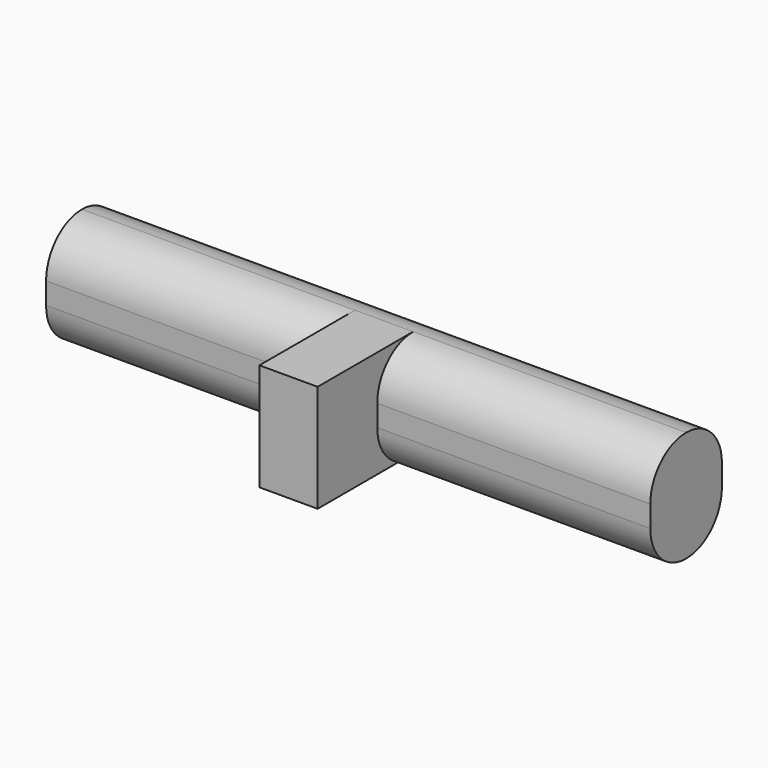
from build123d import *

# Parameters (mm, degrees)
F0_W         = 9.9060004577
F0_H         = 18.2879995555
F1_DEPTH     = 6.35
F2_W         = 9.9060004577
F2_H         = 18.2879995555
F3_DEPTH     = 15.24
F4_T1_DEPTH  = 140.9700014576
F4_T3_DEPTH  = 65.5320005
F4_T5_DEPTH  = 65.5320005
F4_T10_DEPTH = 140.9700014576
F4_T16_DEPTH = 140.9700014576
F4_T22_DEPTH = 140.9700014576
F4_T29_DEPTH = 140.9700014576
F4_T35_DEPTH = 140.9700014576
F4_T41_DEPTH = 84.5820005
F4_T46_DEPTH = 84.5820005


# Not quite as in the source:
# - a fillet or chamfer that OpenCascade refuses, or shapes differently, is made with other operations: its cross-section is extruded or revolved along the edge and cut away or added


with BuildPart() as f1:
    # F0 (on Front) → F1 (new body, symmetric)
    with BuildSketch(Plane.XZ):
        with Locations((-4.9530002289, 9.1439997777)):
            Rectangle(F0_W, F0_H)
    extrude(amount=F1_DEPTH, both=True)

    # F2 (on face) → F3 (join)
    with BuildSketch(Plane(origin=(0, 6.35, 0), x_dir=(-1, 0, 0), z_dir=(0, 1, 0))):
        Polygon((0, 18.2879995555), (-46.4820005, 18.2879995555), (-46.4820005, -0.6095990539), (56.3880009577, -0.6095990539), (56.3880009577, 18.2879995555), (9.9060004577, 18.2879995555), (9.9060004577, 0), (0, 0), align=None)
        with Locations((4.9530002289, 9.1439997777)):
            Rectangle(F2_W, F2_H)
    extrude(amount=F3_DEPTH)

    # F4: fillet of radius 7.62 on 5 edges, made by hand

    # F4_s2 → F4_t1 (cut)
    with BuildSketch(Plane.YZ.offset(-75.4380009577)):
        with BuildLine():
            ThreePointArc((13.97, -0.6095990539), (19.3581536726, 1.6222472735), (21.59, 7.0104009461))
            Line((21.59, 7.0104009461), (21.59, -0.6095990539))
            Line((21.59, -0.6095990539), (13.97, -0.6095990539))
        make_face()
        with BuildLine():
            ThreePointArc((13.97, 18.2879995555), (19.3581536726, 16.0561532281), (21.59, 10.6679995555))
            Line((21.59, 10.6679995555), (21.59, 18.2879995555))
            Line((21.59, 18.2879995555), (13.97, 18.2879995555))
        make_face()
    extrude(amount=F4_T1_DEPTH, mode=Mode.SUBTRACT)

    # F4_s4 → F4_t3 (cut)
    with BuildSketch(Plane.YZ.offset(-75.4380009577)):
        with BuildLine():
            ThreePointArc((13.97, 18.2879995555), (8.5818463274, 16.0561532281), (6.35, 10.6679995555))
            Line((6.35, 10.6679995555), (6.35, 18.2879995555))
            Line((6.35, 18.2879995555), (13.97, 18.2879995555))
        make_face()
    extrude(amount=F4_T3_DEPTH, mode=Mode.SUBTRACT)

    # F4_s6 → F4_t5 (cut)
    with BuildSketch(Plane.YZ):
        with BuildLine():
            ThreePointArc((13.97, 18.2879995555), (8.5818463274, 16.0561532281), (6.35, 10.6679995555))
            Line((6.35, 10.6679995555), (6.35, 18.2879995555))
            Line((6.35, 18.2879995555), (13.97, 18.2879995555))
        make_face()
    extrude(amount=F4_T5_DEPTH, mode=Mode.SUBTRACT)


with BuildPart() as f4_tool8:
    # F4_s9 → F4_t10 (new body)
    with BuildSketch(Plane.YZ.offset(65.5320005)):
        with BuildLine():
            ThreePointArc((13.97, -0.6095990539), (8.5818463274, 1.6222472735), (6.35, 7.0104009461))
            Line((6.35, 7.0104009461), (6.35, -0.6095990539))
            Line((6.35, -0.6095990539), (13.97, -0.6095990539))
        make_face()
    extrude(amount=-F4_T10_DEPTH)

    split(bisect_by=Plane.YZ, keep=Keep.TOP)

    split(bisect_by=Plane.XY, keep=Keep.BOTTOM)


with BuildPart() as f1_1:
    add(f1.part)

    # F4_t7: cut F4_tool8
    add(f4_tool8.part, mode=Mode.SUBTRACT)


with BuildPart() as f4_tool14:
    # F4_s15 → F4_t16 (new body)
    with BuildSketch(Plane.YZ.offset(65.5320005)):
        with BuildLine():
            ThreePointArc((13.97, -0.6095990539), (8.5818463274, 1.6222472735), (6.35, 7.0104009461))
            Line((6.35, 7.0104009461), (6.35, -0.6095990539))
            Line((6.35, -0.6095990539), (13.97, -0.6095990539))
        make_face()
    extrude(amount=-F4_T16_DEPTH)

    split(bisect_by=Plane.YZ, keep=Keep.TOP)

    split(bisect_by=Plane.XY, keep=Keep.TOP)


with BuildPart() as f1_2:
    add(f1_1.part)

    # F4_t13: cut F4_tool14
    add(f4_tool14.part, mode=Mode.SUBTRACT)


with BuildPart() as f4_tool20:
    # F4_s21 → F4_t22 (new body)
    with BuildSketch(Plane.YZ.offset(65.5320005)):
        with BuildLine():
            ThreePointArc((13.97, -0.6095990539), (8.5818463274, 1.6222472735), (6.35, 7.0104009461))
            Line((6.35, 7.0104009461), (6.35, -0.6095990539))
            Line((6.35, -0.6095990539), (13.97, -0.6095990539))
        make_face()
    extrude(amount=-F4_T22_DEPTH)

    split(bisect_by=Plane.YZ, keep=Keep.BOTTOM)

    split(bisect_by=Plane.XY, keep=Keep.BOTTOM)

    split(bisect_by=Plane.YZ.offset(-9.9060004577), keep=Keep.TOP)


with BuildPart() as f1_3:
    add(f1_2.part)

    # F4_t19: cut F4_tool20
    add(f4_tool20.part, mode=Mode.SUBTRACT)


with BuildPart() as f4_tool27:
    # F4_s28 → F4_t29 (new body)
    with BuildSketch(Plane.YZ.offset(65.5320005)):
        with BuildLine():
            ThreePointArc((13.97, -0.6095990539), (8.5818463274, 1.6222472735), (6.35, 7.0104009461))
            Line((6.35, 7.0104009461), (6.35, -0.6095990539))
            Line((6.35, -0.6095990539), (13.97, -0.6095990539))
        make_face()
    extrude(amount=-F4_T29_DEPTH)

    split(bisect_by=Plane.XY, keep=Keep.BOTTOM)

    split(bisect_by=Plane.YZ.offset(-9.9060004577), keep=Keep.BOTTOM)


with BuildPart() as f1_4:
    add(f1_3.part)

    # F4_t26: cut F4_tool27
    add(f4_tool27.part, mode=Mode.SUBTRACT)


with BuildPart() as f4_tool33:
    # F4_s34 → F4_t35 (new body)
    with BuildSketch(Plane.YZ.offset(65.5320005)):
        with BuildLine():
            ThreePointArc((13.97, -0.6095990539), (8.5818463274, 1.6222472735), (6.35, 7.0104009461))
            Line((6.35, 7.0104009461), (6.35, -0.6095990539))
            Line((6.35, -0.6095990539), (13.97, -0.6095990539))
        make_face()
    extrude(amount=-F4_T35_DEPTH)

    split(bisect_by=Plane.XY, keep=Keep.TOP)

    split(bisect_by=Plane.YZ.offset(-9.9060004577), keep=Keep.BOTTOM)


with BuildPart() as f1_5:
    add(f1_4.part)

    # F4_t32: cut F4_tool33
    add(f4_tool33.part, mode=Mode.SUBTRACT)


with BuildPart() as f4_tool39:
    # F4_s40 → F4_t41 (new body)
    with BuildSketch(Plane.YZ.offset(-75.4380009577)):
        with BuildLine():
            ThreePointArc((13.97, 18.2879995555), (8.5818463274, 16.0561532281), (6.35, 10.6679995555))
            Line((6.35, 10.6679995555), (6.35, 18.2879995555))
            Line((6.35, 18.2879995555), (13.97, 18.2879995555))
        make_face()
    extrude(amount=F4_T41_DEPTH)

    split(bisect_by=Plane.YZ, keep=Keep.TOP)


with BuildPart() as f1_6:
    add(f1_5.part)

    # F4_t38: cut F4_tool39
    add(f4_tool39.part, mode=Mode.SUBTRACT)


with BuildPart() as f4_tool44:
    # F4_s45 → F4_t46 (new body)
    with BuildSketch(Plane.YZ.offset(-19.05)):
        with BuildLine():
            ThreePointArc((13.97, 18.2879995555), (8.5818463274, 16.0561532281), (6.35, 10.6679995555))
            Line((6.35, 10.6679995555), (6.35, 18.2879995555))
            Line((6.35, 18.2879995555), (13.97, 18.2879995555))
        make_face()
    extrude(amount=F4_T46_DEPTH)

    split(bisect_by=Plane.YZ.offset(-9.9060004577), keep=Keep.BOTTOM)


with BuildPart() as f1_7:
    add(f1_6.part)

    # F4_t43: cut F4_tool44
    add(f4_tool44.part, mode=Mode.SUBTRACT)


solid = f1_7.part
